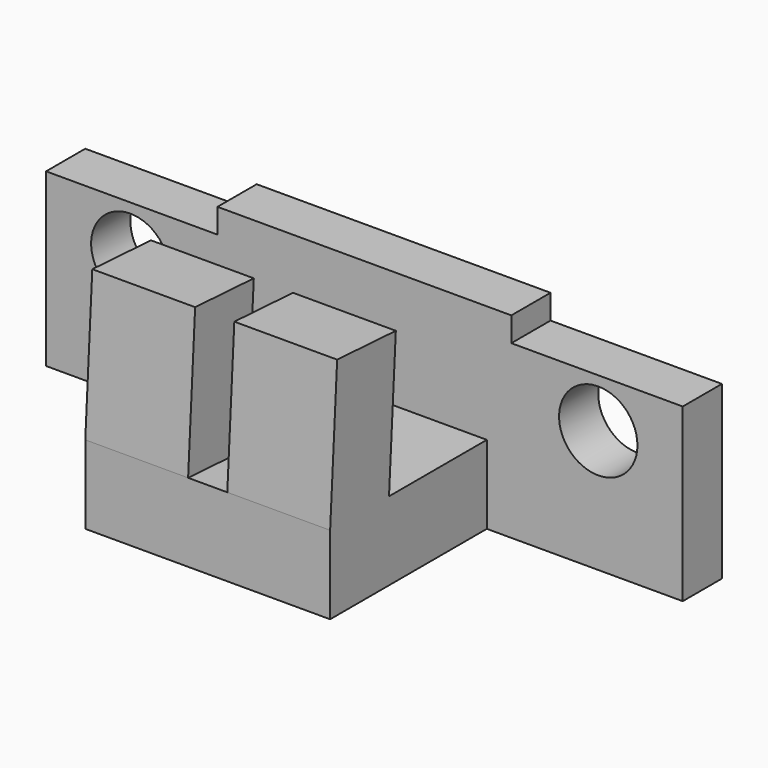
from build123d import *

# Parameters (mm, degrees)
F0_R     = 2.032
F1_DEPTH = 2.54
F2_W     = 12.7
F2_H     = 4.064
F3_DEPTH = 10.16
F5_DEPTH = 12.7
F6_W     = 2.032
F6_H     = 7.62
F7_DEPTH = 3.81


with BuildPart() as f1:
    # F0 (on Front) → F1 (new body)
    with BuildSketch(Plane.XZ):
        Polygon((7.62, 3.81), (-7.62, 3.81), (-7.62, 2.54), (-16.51, 2.54), (-16.51, -6.35), (16.51, -6.35), (16.51, 2.54), (7.62, 2.54), align=None)
        with Locations((-12.1412, 0)):
            Circle(F0_R, mode=Mode.SUBTRACT)
        with Locations((12.1285, 0)):
            Circle(F0_R, mode=Mode.SUBTRACT)
    extrude(amount=F1_DEPTH)

    # F2 (on face) → F3 (join)
    with BuildSketch(Plane.XZ.offset(2.54)):
        with Locations((0, -4.318)):
            Rectangle(F2_W, F2_H)
    extrude(amount=F3_DEPTH)

    # F4 (on face) → F5 (join)
    with BuildSketch(Plane(origin=(-6.35, 0, 0), x_dir=(0, -1, 0), z_dir=(-1, 0, 0))):
        Polygon((8.8831661625, -2.286), (12.7, -2.286), (12.2442190351, 5.3203567963), (8.441040637, 5.0924663138), align=None)
    extrude(amount=-F5_DEPTH)

    # F6 (on face) → F7 (cut)
    with BuildSketch(Plane(origin=(0, -12.5180738926, 0.7500962617), x_dir=(1, 0, 0), z_dir=(0, -0.9982095533, 0.0598137749))):
        with Locations((0, 0.7684580196)):
            Rectangle(F6_W, F6_H)
    extrude(amount=-F7_DEPTH, mode=Mode.SUBTRACT)


solid = f1.part
